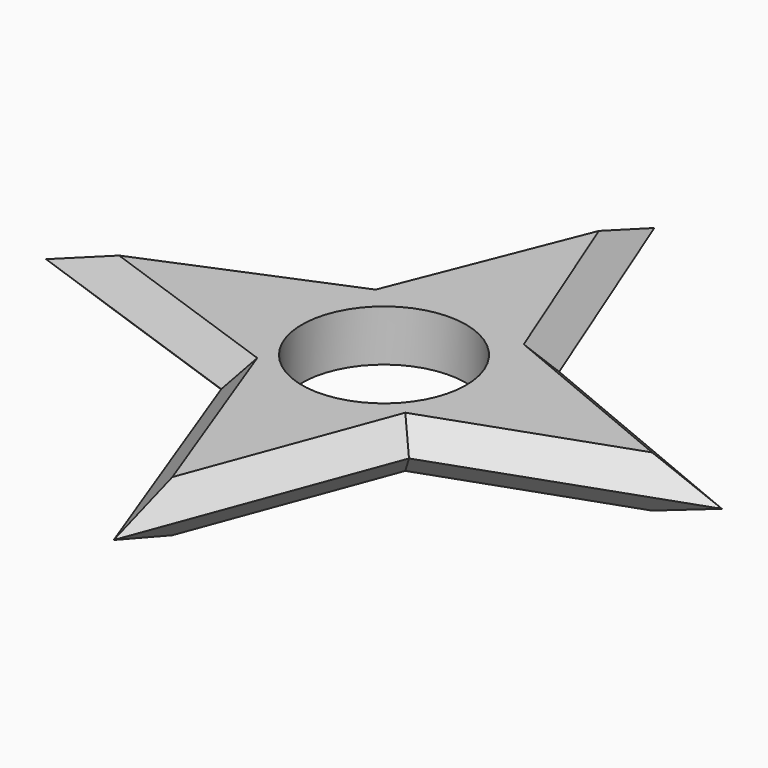
from build123d import *

# Parameters (mm, degrees)
F0_R     = 11.0998
F1_DEPTH = 6.9342
F2_SIZE  = 3.4671
F3_SIZE  = 3.46709


# Not quite as in the source:
# - a fillet or chamfer is up to 0.001 mm smaller than in the source, because OpenCascade refuses the exact size


with BuildPart() as f1:
    # F0 (on Top) → F1 (new body)
    with BuildSketch(Plane.XY):
        Polygon((12.7, 13.7528510513), (0, 45.72), (-12.7, 13.7528510513), (-45.72, 0), (-12.7, -11.6471489487), (0, -45.72), (12.7, -11.6471489487), (45.72, 0), align=None)
        Circle(F0_R, mode=Mode.SUBTRACT)
    extrude(amount=F1_DEPTH)

    # F2
    f2_edges = [f1.edges().sort_by_distance(p)[0] for p in [
        (6.35, -28.683574, 6.9342),
        (29.21, -5.823574, 6.9342),
        (-29.21, -5.823574, 6.9342),
        (-6.35, 29.736426, 6.9342),
        (-29.21, 6.876426, 6.9342),
        (6.35, 29.736426, 6.9342),
        (29.21, 6.876426, 6.9342),
        (-6.35, -28.683574, 6.9342),
    ]]
    chamfer(f2_edges, length=F2_SIZE)

    # F3 (size 3.4671 in the source; OpenCascade refuses exactly that, so slightly less here)
    f3_edges = [f1.edges().sort_by_distance(p)[0] for p in [
        (6.35, -28.683574, 0),
        (29.21, -5.823574, 0),
        (-29.21, -5.823574, 0),
        (-6.35, -28.683574, 0),
        (6.35, 29.736426, 0),
        (29.21, 6.876426, 0),
        (-29.21, 6.876426, 0),
        (-6.35, 29.736426, 0),
    ]]
    chamfer(f3_edges, length=F3_SIZE)


solid = f1.part
